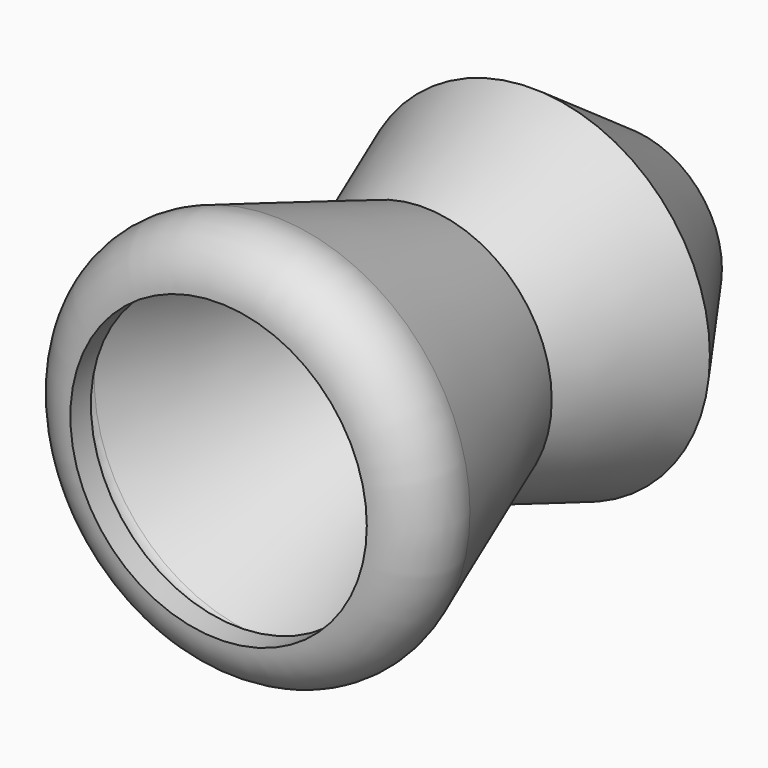
from build123d import *

# Parameters (mm, degrees)
F0_R     = 63.5
F1_DEPTH = 127
F1_TAPER = -20
F2_R     = 25.4
F3_SIZE  = 63.5
F4_T     = -12.7


# Not quite as in the source:
# - a shell that OpenCascade refuses in one call is made with other operations: the cavity is built on its own and cut out


with BuildPart() as f1:
    # F0 (on Front) → F1 (new body, symmetric)
    with BuildSketch(Plane.XZ):
        Circle(F0_R)
    extrude(amount=F1_DEPTH, both=True, taper=F1_TAPER)

    # F2
    f2_edges = [f1.edges().sort_by_distance(p)[0] for p in [
        (-109.72422, -127, 0),
    ]]
    fillet(f2_edges, radius=F2_R)

    # F3
    f3_edges = [f1.edges().sort_by_distance(p)[0] for p in [
        (-109.72422, 127, 0),
    ]]
    chamfer(f3_edges, length=F3_SIZE)

    # F4: a shell. OpenCascade refuses it in one call, so the cavity is built on its own and cut out:
    # the body offset inwards by the wall thickness, plus a prism from it out through each open face.
    f4_core = offset(f1.part, amount=F4_T, kind=Kind.INTERSECTION, mode=Mode.PRIVATE)
    f4_exits = [f4_core.faces().sort_by_distance(p)[0] for p in [
        (0, -114.3, 0),
    ]]
    add(f4_core, mode=Mode.SUBTRACT)
    extrude(f4_exits, amount=-F4_T, mode=Mode.SUBTRACT)


solid = f1.part
